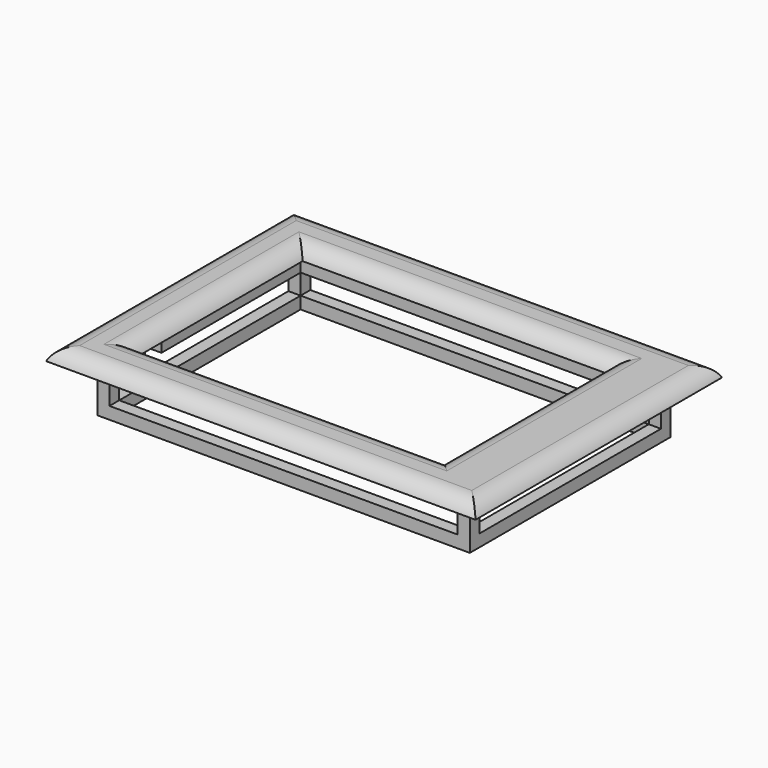
from build123d import *

# Parameters (mm, degrees)
F2_W          = 105.7
F2_H          = 75.8
F2_W_2        = 8
F2_H_2        = 2.5
F2_H_3        = 50.8
F4_DEPTH      = 3
F3_W          = 91.7
F3_H          = 61.8
F3_W_2        = 85.7
F3_H_2        = 55.8
F5_DEPTH      = 12.3
F6_W          = 85.7
F6_H          = 5
F7_DEPTH      = 50.4239358673
F7_DEPTH_BACK = 25
F9_DEPTH      = 68.6133680484
F9_DEPTH_BACK = 37.0886319516
F10_T1_DEPTH  = 98.7128784748
F10_T3_DEPTH  = 128.6128784748
F10_T5_DEPTH  = 50.8
F10_T7_DEPTH  = 75.2
F10_T13_DEPTH = 62.2564392374
F10_T17_DEPTH = 86.6564392374
F10_T24_DEPTH = 86.6564392374
F10_T28_DEPTH = 62.2564392374
F10_T35_DEPTH = 86.6564392374
F10_T39_DEPTH = 62.2564392374
F10_T46_DEPTH = 86.6564392374
F10_T50_DEPTH = 62.2564392374


# Not quite as in the source:
# - a fillet or chamfer that OpenCascade refuses, or shapes differently, is made with other operations: its cross-section is extruded or revolved along the edge and cut away or added


with BuildPart() as f4:
    # F2 (on Top) → F4 (new body)
    with BuildSketch(Plane.XY):
        with Locations((-15.7623680484, 12.5229358673)):
            Rectangle(F2_W, F2_H)
        Polygon((-58.6123680484, -15.3770641327), (-58.6123680484, 40.4229358673), (19.0876319516, 40.4229358673), (27.0876319516, 40.4229358673), (27.0876319516, 37.9229358673), (27.0876319516, -12.8770641327), (27.0876319516, -15.3770641327), (19.0876319516, -15.3770641327), align=None, mode=Mode.SUBTRACT)
        Polygon((19.0876319516, 40.4229358673), (-58.6123680484, 40.4229358673), (-58.6123680484, -15.3770641327), (19.0876319516, -15.3770641327), (19.0876319516, -12.8770641327), (-56.1123680484, -12.8770641327), (-56.1123680484, 37.9229358673), (19.0876319516, 37.9229358673), align=None)
        with Locations((23.0876319516, 39.1729358673)):
            Rectangle(F2_W_2, F2_H_2)
        with Locations((23.0876319516, 12.5229358673)):
            Rectangle(F2_W_2, F2_H_3)
        with Locations((23.0876319516, -14.1270641327)):
            Rectangle(F2_W_2, F2_H_2)
    extrude(amount=F4_DEPTH)

    # F3 (on Top) → F5 (join)
    with BuildSketch(Plane.XY):
        with Locations((-15.7623680484, 12.5229358673)):
            Rectangle(F3_W, F3_H)
        with Locations((-15.7623680484, 12.5229358673)):
            Rectangle(F3_W_2, F3_H_2, mode=Mode.SUBTRACT)
    extrude(amount=-F5_DEPTH)

    # F6 (on Front) → F7 (cut, two sides)
    with BuildSketch(Plane.XZ) as f7_sk:
        with Locations((-15.7623680484, -6.8)):
            Rectangle(F6_W, F6_H)
    extrude(amount=-F7_DEPTH, mode=Mode.SUBTRACT)
    extrude(f7_sk.sketch, amount=F7_DEPTH_BACK, mode=Mode.SUBTRACT)

    # F8 (on Right) → F9 (cut, two sides)
    with BuildSketch(Plane.YZ) as f9_sk:
        Polygon((-2.3770641327, -3.112567123), (-2.3770641327, 0), (-7.3770641327, 0), (-7.3770641327, -3.112567123), (-7.3770641327, -4.3), (-2.3770641327, -4.3), align=None)
        Polygon((40.4229358673, -9.3), (40.4229358673, -4.3), (-2.3770641327, -4.3), (-7.3770641327, -4.3), (-15.3770641327, -4.3), (-15.3770641327, -9.3), align=None)
    extrude(amount=-F9_DEPTH, mode=Mode.SUBTRACT)
    extrude(f9_sk.sketch, amount=F9_DEPTH_BACK, mode=Mode.SUBTRACT)

    # F10: fillet of radius 5 on 8 edges, made by hand

    # F10_s2 → F10_t1 (cut)
    with BuildSketch(Plane.XZ.offset(-61.8793751047)):
        with BuildLine():
            ThreePointArc((37.0876319516, 0), (35.2436690442, 2.1833001327), (32.5050562567, 3))
            Line((32.5050562567, 3), (32.5050562567, 3.1))
            Line((32.5050562567, 3.1), (37.0876319516, 3.1))
            Line((37.0876319516, 3.1), (37.1876319516, 3))
            ThreePointArc((37.1876319516, 3), (37.1876319516, 1.5), (37.1792834655, 0.04))
            Line((37.1792834655, 0.04), (37.0876319516, 0))
        make_face()
        with BuildLine():
            ThreePointArc((-68.6123680484, 0), (-66.768405141, 2.1833001327), (-64.0297923534, 3))
            Line((-64.0297923534, 3), (-64.0297923534, 3.1))
            Line((-64.0297923534, 3.1), (-68.6123680484, 3.1))
            Line((-68.6123680484, 3.1), (-68.7123680484, 3))
            ThreePointArc((-68.7123680484, 3), (-68.7123680484, 1.5), (-68.7040195623, 0.04))
            Line((-68.7040195623, 0.04), (-68.6123680484, 0))
        make_face()
    extrude(amount=F10_T1_DEPTH, mode=Mode.SUBTRACT)

    # F10_s4 → F10_t3 (cut)
    with BuildSketch(Plane.YZ.offset(-80.0688072858)):
        with BuildLine():
            ThreePointArc((50.4229358673, 0), (48.5789729599, 2.1833001327), (45.8403601724, 3))
            Line((45.8403601724, 3), (45.8403601724, 3.1))
            Line((45.8403601724, 3.1), (50.4229358673, 3.1))
            Line((50.4229358673, 3.1), (50.5229358673, 3))
            ThreePointArc((50.5229358673, 3), (50.5229358673, 1.5), (50.5145873812, 0.04))
            Line((50.5145873812, 0.04), (50.4229358673, 0))
        make_face()
        with BuildLine():
            ThreePointArc((-20.7944884377, 3), (-23.5331012253, 2.1833001327), (-25.3770641327, 0))
            Line((-25.3770641327, 0), (-25.4687156466, 0.04))
            ThreePointArc((-25.4687156466, 0.04), (-25.4770641327, 1.5), (-25.4770641327, 3))
            Line((-25.4770641327, 3), (-25.3770641327, 3.1))
            Line((-25.3770641327, 3.1), (-20.7944884377, 3.1))
            Line((-20.7944884377, 3.1), (-20.7944884377, 3))
        make_face()
    extrude(amount=F10_T3_DEPTH, mode=Mode.SUBTRACT)

    # F10_s6 → F10_t5 (cut)
    with BuildSketch(Plane.XZ.offset(-37.9229358673)):
        with BuildLine():
            ThreePointArc((19.0876319516, 0), (20.931594859, 2.1833001327), (23.6702076466, 3))
            Line((23.6702076466, 3), (23.6702076466, 3.1))
            Line((23.6702076466, 3.1), (19.0876319516, 3.1))
            Line((19.0876319516, 3.1), (18.9876319516, 3))
            ThreePointArc((18.9876319516, 3), (18.9876319516, 1.5), (18.9959804377, 0.04))
            Line((18.9959804377, 0.04), (19.0876319516, 0))
        make_face()
        with BuildLine():
            ThreePointArc((-56.1123680484, 0), (-57.9563309558, 2.1833001327), (-60.6949437433, 3))
            Line((-60.6949437433, 3), (-60.6949437433, 3.1))
            Line((-60.6949437433, 3.1), (-56.1123680484, 3.1))
            Line((-56.1123680484, 3.1), (-56.0123680484, 3))
            ThreePointArc((-56.0123680484, 3), (-56.0123680484, 1.5), (-56.0207165345, 0.04))
            Line((-56.0207165345, 0.04), (-56.1123680484, 0))
        make_face()
    extrude(amount=F10_T5_DEPTH, mode=Mode.SUBTRACT)

    # F10_s8 → F10_t7 (cut)
    with BuildSketch(Plane.YZ.offset(-56.1123680484)):
        with BuildLine():
            ThreePointArc((-12.8770641327, 0), (-14.7210270401, 2.1833001327), (-17.4596398276, 3))
            Line((-17.4596398276, 3), (-17.4596398276, 3.1))
            Line((-17.4596398276, 3.1), (-12.8770641327, 3.1))
            Line((-12.8770641327, 3.1), (-12.7770641327, 3))
            ThreePointArc((-12.7770641327, 3), (-12.7770641327, 1.5), (-12.7854126188, 0.04))
            Line((-12.7854126188, 0.04), (-12.8770641327, 0))
        make_face()
        with BuildLine():
            ThreePointArc((37.9229358673, 0), (39.7668987747, 2.1833001327), (42.5055115623, 3))
            Line((42.5055115623, 3), (42.5055115623, 3.1))
            Line((42.5055115623, 3.1), (37.9229358673, 3.1))
            Line((37.9229358673, 3.1), (37.8229358673, 3))
            ThreePointArc((37.8229358673, 3), (37.8229358673, 1.5), (37.8312843534, 0.04))
            Line((37.8312843534, 0.04), (37.9229358673, 0))
        make_face()
    extrude(amount=F10_T7_DEPTH, mode=Mode.SUBTRACT)


with BuildPart() as f10_tool11:
    # F10_s12 → F10_t13 (new body)
    with BuildSketch(Plane.XZ.offset(-49.3793751047)):
        with BuildLine():
            ThreePointArc((19.0876319516, 0), (20.931594859, 2.1833001327), (23.6702076466, 3))
            Line((23.6702076466, 3), (23.6702076466, 3.1))
            Line((23.6702076466, 3.1), (19.0876319516, 3.1))
            Line((19.0876319516, 3.1), (18.9876319516, 3))
            ThreePointArc((18.9876319516, 3), (18.9876319516, 1.5), (18.9959804377, 0.04))
            Line((18.9959804377, 0.04), (19.0876319516, 0))
        make_face()
    extrude(amount=F10_T13_DEPTH)

    split(bisect_by=Plane.XZ.offset(-37.9229358673), keep=Keep.BOTTOM)


with BuildPart() as f10_tool15:
    # F10_s16 → F10_t17 (new body)
    with BuildSketch(Plane.YZ.offset(-56.1123680484)):
        with BuildLine():
            ThreePointArc((37.9229358673, 0), (39.7668987747, 2.1833001327), (42.5055115623, 3))
            Line((42.5055115623, 3), (42.5055115623, 3.1))
            Line((42.5055115623, 3.1), (37.9229358673, 3.1))
            Line((37.9229358673, 3.1), (37.8229358673, 3))
            ThreePointArc((37.8229358673, 3), (37.8229358673, 1.5), (37.8312843534, 0.04))
            Line((37.8312843534, 0.04), (37.9229358673, 0))
        make_face()
    extrude(amount=F10_T17_DEPTH)

    split(bisect_by=Plane.YZ.offset(19.0876319516), keep=Keep.TOP)


with BuildPart() as f10_tool11_1:
    add(f10_tool11.part)

    # F10_t19: intersect F10_tool15
    add(f10_tool15.part, mode=Mode.INTERSECT)


with BuildPart() as f4_1:
    add(f4.part)

    # F10_t9: cut F10_tool11
    add(f10_tool11_1.part, mode=Mode.SUBTRACT)


with BuildPart() as f10_tool22:
    # F10_s23 → F10_t24 (new body)
    with BuildSketch(Plane.YZ.offset(30.544071189)):
        with BuildLine():
            ThreePointArc((-12.8770641327, 0), (-14.7210270401, 2.1833001327), (-17.4596398276, 3))
            Line((-17.4596398276, 3), (-17.4596398276, 3.1))
            Line((-17.4596398276, 3.1), (-12.8770641327, 3.1))
            Line((-12.8770641327, 3.1), (-12.7770641327, 3))
            ThreePointArc((-12.7770641327, 3), (-12.7770641327, 1.5), (-12.7854126188, 0.04))
            Line((-12.7854126188, 0.04), (-12.8770641327, 0))
        make_face()
    extrude(amount=-F10_T24_DEPTH)

    split(bisect_by=Plane.YZ.offset(19.0876319516), keep=Keep.TOP)


with BuildPart() as f10_tool26:
    # F10_s27 → F10_t28 (new body)
    with BuildSketch(Plane.XZ.offset(-37.9229358673)):
        with BuildLine():
            ThreePointArc((19.0876319516, 0), (20.931594859, 2.1833001327), (23.6702076466, 3))
            Line((23.6702076466, 3), (23.6702076466, 3.1))
            Line((23.6702076466, 3.1), (19.0876319516, 3.1))
            Line((19.0876319516, 3.1), (18.9876319516, 3))
            ThreePointArc((18.9876319516, 3), (18.9876319516, 1.5), (18.9959804377, 0.04))
            Line((18.9959804377, 0.04), (19.0876319516, 0))
        make_face()
    extrude(amount=F10_T28_DEPTH)

    split(bisect_by=Plane.XZ.offset(12.8770641327), keep=Keep.TOP)


with BuildPart() as f10_tool22_1:
    add(f10_tool22.part)

    # F10_t30: intersect F10_tool26
    add(f10_tool26.part, mode=Mode.INTERSECT)


with BuildPart() as f4_2:
    add(f4_1.part)

    # F10_t20: cut F10_tool22
    add(f10_tool22_1.part, mode=Mode.SUBTRACT)


with BuildPart() as f10_tool33:
    # F10_s34 → F10_t35 (new body)
    with BuildSketch(Plane.YZ.offset(19.0876319516)):
        with BuildLine():
            ThreePointArc((-12.8770641327, 0), (-14.7210270401, 2.1833001327), (-17.4596398276, 3))
            Line((-17.4596398276, 3), (-17.4596398276, 3.1))
            Line((-17.4596398276, 3.1), (-12.8770641327, 3.1))
            Line((-12.8770641327, 3.1), (-12.7770641327, 3))
            ThreePointArc((-12.7770641327, 3), (-12.7770641327, 1.5), (-12.7854126188, 0.04))
            Line((-12.7854126188, 0.04), (-12.8770641327, 0))
        make_face()
    extrude(amount=-F10_T35_DEPTH)

    split(bisect_by=Plane.YZ.offset(-56.1123680484), keep=Keep.BOTTOM)


with BuildPart() as f10_tool37:
    # F10_s38 → F10_t39 (new body)
    with BuildSketch(Plane.XZ.offset(24.3335033701)):
        with BuildLine():
            ThreePointArc((-56.1123680484, 0), (-57.9563309558, 2.1833001327), (-60.6949437433, 3))
            Line((-60.6949437433, 3), (-60.6949437433, 3.1))
            Line((-60.6949437433, 3.1), (-56.1123680484, 3.1))
            Line((-56.1123680484, 3.1), (-56.0123680484, 3))
            ThreePointArc((-56.0123680484, 3), (-56.0123680484, 1.5), (-56.0207165345, 0.04))
            Line((-56.0207165345, 0.04), (-56.1123680484, 0))
        make_face()
    extrude(amount=-F10_T39_DEPTH)

    split(bisect_by=Plane.XZ.offset(12.8770641327), keep=Keep.TOP)


with BuildPart() as f10_tool33_1:
    add(f10_tool33.part)

    # F10_t41: intersect F10_tool37
    add(f10_tool37.part, mode=Mode.INTERSECT)


with BuildPart() as f4_3:
    add(f4_2.part)

    # F10_t31: cut F10_tool33
    add(f10_tool33_1.part, mode=Mode.SUBTRACT)


with BuildPart() as f10_tool44:
    # F10_s45 → F10_t46 (new body)
    with BuildSketch(Plane.YZ.offset(-67.5688072858)):
        with BuildLine():
            ThreePointArc((37.9229358673, 0), (39.7668987747, 2.1833001327), (42.5055115623, 3))
            Line((42.5055115623, 3), (42.5055115623, 3.1))
            Line((42.5055115623, 3.1), (37.9229358673, 3.1))
            Line((37.9229358673, 3.1), (37.8229358673, 3))
            ThreePointArc((37.8229358673, 3), (37.8229358673, 1.5), (37.8312843534, 0.04))
            Line((37.8312843534, 0.04), (37.9229358673, 0))
        make_face()
    extrude(amount=F10_T46_DEPTH)

    split(bisect_by=Plane.YZ.offset(-56.1123680484), keep=Keep.BOTTOM)


with BuildPart() as f10_tool48:
    # F10_s49 → F10_t50 (new body)
    with BuildSketch(Plane.XZ.offset(12.8770641327)):
        with BuildLine():
            ThreePointArc((-56.1123680484, 0), (-57.9563309558, 2.1833001327), (-60.6949437433, 3))
            Line((-60.6949437433, 3), (-60.6949437433, 3.1))
            Line((-60.6949437433, 3.1), (-56.1123680484, 3.1))
            Line((-56.1123680484, 3.1), (-56.0123680484, 3))
            ThreePointArc((-56.0123680484, 3), (-56.0123680484, 1.5), (-56.0207165345, 0.04))
            Line((-56.0207165345, 0.04), (-56.1123680484, 0))
        make_face()
    extrude(amount=-F10_T50_DEPTH)

    split(bisect_by=Plane.XZ.offset(-37.9229358673), keep=Keep.BOTTOM)


with BuildPart() as f10_tool44_1:
    add(f10_tool44.part)

    # F10_t52: intersect F10_tool48
    add(f10_tool48.part, mode=Mode.INTERSECT)


with BuildPart() as f4_4:
    add(f4_3.part)

    # F10_t42: cut F10_tool44
    add(f10_tool44_1.part, mode=Mode.SUBTRACT)


solid = f4_4.part
